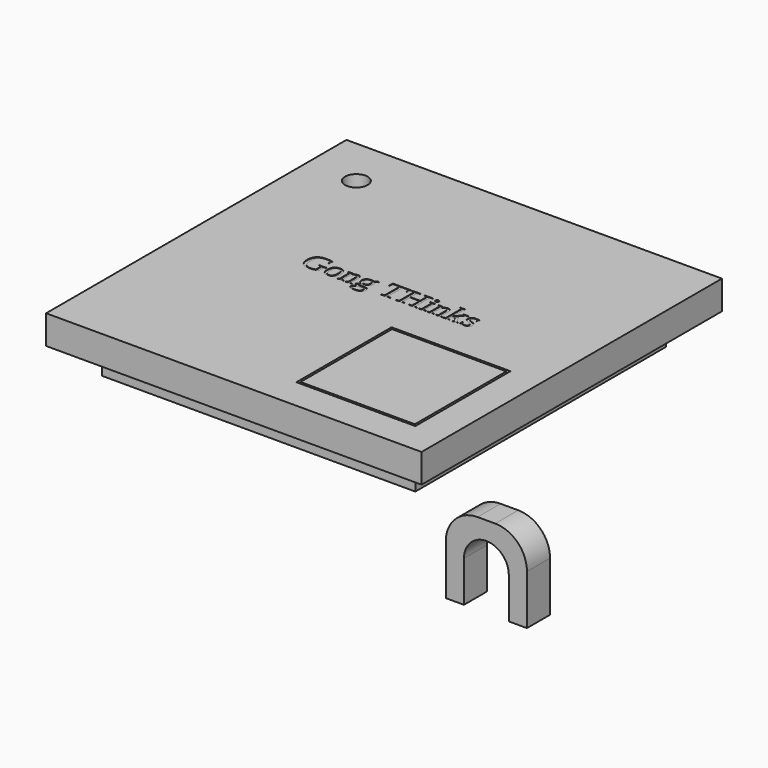
from build123d import *

# Parameters (mm, degrees)
F1_W        = 69
F1_H        = 69
F1_W_2      = 20.186291501
F1_H_2      = 20.186291501
F1_R        = 2.5
F2_DEPTH    = 6.35
F3_DEPTH    = 6.25
F4_W        = 9.8855943071
F4_H        = 4
F5_DEPTH    = 6.35
F6_R        = 7
F7_R        = 7
F8_R        = 5
F9_T1_DEPTH = 6.35
F0_W        = 82.7
F0_H        = 82.7
F0_W_2      = 26.19
F0_H_2      = 26.19
F10_DEPTH   = 6.35
F11_DEPTH   = 6.35
F0_W_3      = 25.19
F0_H_3      = 25.19
F12_DEPTH   = 6.35


# Not quite as in the source:
# - a fillet or chamfer that OpenCascade refuses, or shapes differently, is made with other operations: its cross-section is extruded or revolved along the edge and cut away or added


with BuildPart() as f2:
    # F1 (on Top) → F2 (new body)
    with BuildSketch(Plane.XY):
        Rectangle(F1_W, F1_H)
        with Locations((21.4068542495, -21.4068542495)):
            Rectangle(F1_W_2, F1_H_2, mode=Mode.SUBTRACT)
        with Locations((-30.5, 30.5)):
            Circle(F1_R, mode=Mode.SUBTRACT)
    extrude(amount=-F2_DEPTH)

    # F0 (on Top) → F3 (join)
    with BuildSketch(Plane.XY):
        with BuildLine():
            add(Edge.make_bspline(
                [(18.7366319096, 0.8951822917), (18.7366319096, 0.4210069444), (18.4366102082, 0.1763237847)],
                knots=[0, 0, 0, 1, 1, 1], degree=2))
            add(Edge.make_bspline(
                [(18.6774956249, 1.2548828125), (18.7366319096, 1.1089409722), (18.7366319096, 0.8951822917)],
                knots=[0, 0, 0, 1, 1, 1], degree=2))
            add(Edge.make_bspline(
                [(18.5114799999, 1.5142144097), (18.6183593401, 1.4008246528), (18.6774956249, 1.2548828125)],
                knots=[0, 0, 0, 1, 1, 1], degree=2))
            add(Edge.make_bspline(
                [(18.2521484026, 1.7057291667), (18.4046006596, 1.6276041667), (18.5114799999, 1.5142144097)],
                knots=[0, 0, 0, 1, 1, 1], degree=2))
            add(Edge.make_bspline(
                [(17.6016492707, 1.953125), (18.0996961457, 1.7838541667), (18.2521484026, 1.7057291667)],
                knots=[0, 0, 0, 1, 1, 1], degree=2))
            add(Edge.make_bspline(
                [(17.2061414582, 2.1733940972), (17.3368923263, 2.041015625), (17.6016492707, 1.953125)],
                knots=[0, 0, 0, 1, 1, 1], degree=2))
            add(Edge.make_bspline(
                [(17.0753905901, 2.4989149306), (17.0753905901, 2.3057725694), (17.2061414582, 2.1733940972)],
                knots=[0, 0, 0, 1, 1, 1], degree=2))
            add(Edge.make_bspline(
                [(17.2197048263, 2.8656684028), (17.0753905901, 2.7300347222), (17.0753905901, 2.4989149306)],
                knots=[0, 0, 0, 1, 1, 1], degree=2))
            add(Edge.make_bspline(
                [(17.6385416318, 3.0013020833), (17.3640190624, 3.0013020833), (17.2197048263, 2.8656684028)],
                knots=[0, 0, 0, 1, 1, 1], degree=2))
            add(Edge.make_bspline(
                [(18.2049478818, 2.841796875), (18.024826354, 3.0013020833), (17.6385416318, 3.0013020833)],
                knots=[0, 0, 0, 1, 1, 1], degree=2))
            Line((18.2049478818, 2.841796875), (18.347091979, 2.4717881944))
            Line((18.347091979, 2.4717881944), (18.5065971874, 2.4717881944))
            Line((18.5065971874, 2.4717881944), (18.5065971874, 3.1673177083))
            add(Edge.make_bspline(
                [(17.6320312151, 3.2725694444), (17.9814235763, 3.2725694444), (18.5065971874, 3.1673177083)],
                knots=[0, 0, 0, 1, 1, 1], degree=2))
            add(Edge.make_bspline(
                [(16.8572916318, 3.0300564236), (17.1437499651, 3.2725694444), (17.6320312151, 3.2725694444)],
                knots=[0, 0, 0, 1, 1, 1], degree=2))
            add(Edge.make_bspline(
                [(16.5708332985, 2.3665364583), (16.5708332985, 2.7875434028), (16.8572916318, 3.0300564236)],
                knots=[0, 0, 0, 1, 1, 1], degree=2))
            add(Edge.make_bspline(
                [(16.6554687151, 1.9618055556), (16.5708332985, 2.1299913194), (16.5708332985, 2.3665364583)],
                knots=[0, 0, 0, 1, 1, 1], degree=2))
            add(Edge.make_bspline(
                [(16.8958115971, 1.6786024306), (16.7401041318, 1.7936197917), (16.6554687151, 1.9618055556)],
                knots=[0, 0, 0, 1, 1, 1], degree=2))
            add(Edge.make_bspline(
                [(17.3944010068, 1.4518229167), (17.0515190624, 1.5635850694), (16.8958115971, 1.6786024306)],
                knots=[0, 0, 0, 1, 1, 1], degree=2))
            Line((17.3944010068, 1.4518229167), (17.6960503124, 1.3530815972))
            add(Edge.make_bspline(
                [(18.2147135068, 0.7628038194), (18.2147135068, 1.1762152778), (17.6960503124, 1.3530815972)],
                knots=[0, 0, 0, 1, 1, 1], degree=2))
            add(Edge.make_bspline(
                [(17.5571614235, 0.1996527778), (18.2147135068, 0.1996527778), (18.2147135068, 0.7628038194)],
                knots=[0, 0, 0, 1, 1, 1], degree=2))
            add(Edge.make_bspline(
                [(16.8963541318, 0.4307725694), (17.1502603818, 0.1996527778), (17.5571614235, 0.1996527778)],
                knots=[0, 0, 0, 1, 1, 1], degree=2))
            Line((16.8963541318, 0.4307725694), (16.7292534374, 0.8745659722))
            Line((16.7292534374, 0.8745659722), (16.5773437151, 0.8745659722))
            Line((16.5773437151, 0.8745659722), (16.5773437151, 0.0911458333))
            add(Edge.make_bspline(
                [(17.0265624651, -0.0189887153), (16.7401041318, 0.0303819444), (16.5773437151, 0.0911458333)],
                knots=[0, 0, 0, 1, 1, 1], degree=2))
            add(Edge.make_bspline(
                [(17.5506510068, -0.068359375), (17.3130207985, -0.068359375), (17.0265624651, -0.0189887153)],
                knots=[0, 0, 0, 1, 1, 1], degree=2))
            add(Edge.make_bspline(
                [(18.4366102082, 0.1763237847), (18.1365885068, -0.068359375), (17.5506510068, -0.068359375)],
                knots=[0, 0, 0, 1, 1, 1], degree=2))
        make_face()
        Polygon((15.2850260068, 2.9437934028), (13.9796874651, 1.5364583333), (13.9796874651, 4.8187934028), (12.9456162846, 4.8187934028), (12.9456162846, 4.6657986111), (13.4165364235, 4.5844184028), (13.4165364235, 0.2376302083), (13.0128905901, 0.1529947917), (13.0128905901, 0), (14.3193142013, 0), (14.3193142013, 0.1529947917), (13.9796874651, 0.2376302083), (13.9796874651, 1.1534288194), (14.3963541318, 1.6102430556), (15.2720051735, 0.2376302083), (14.9801214929, 0.1529947917), (14.9801214929, 0), (16.2854600346, 0), (16.2854600346, 0.1529947917), (15.9393228818, 0.2311197917), (14.772873229, 2.0279947917), (15.6821614235, 2.9568142361), (16.0782117707, 3.0349392361), (16.0782117707, 3.1879340278), (14.9529947568, 3.1879340278), (14.9529947568, 3.0349392361), align=None)
        with BuildLine():
            add(Edge.make_bspline(
                [(10.4401909374, 2.9296875), (10.700607604, 3.0794270833), (10.9957464929, 3.1759982639)],
                knots=[0, 0, 0, 1, 1, 1], degree=2))
            Line((10.4401909374, 2.9296875), (10.4087239235, 3.1879340278))
            Line((10.4087239235, 3.1879340278), (9.5005207985, 3.1879340278))
            Line((9.5005207985, 3.1879340278), (9.5005207985, 3.0349392361))
            Line((9.5005207985, 3.0349392361), (9.8835503124, 2.9503038194))
            Line((9.8835503124, 2.9503038194), (9.8835503124, 0.2376302083))
            Line((9.8835503124, 0.2376302083), (9.5005207985, 0.1529947917))
            Line((9.5005207985, 0.1529947917), (9.5005207985, 0))
            Line((9.5005207985, 0), (10.8774739235, 0))
            Line((10.8774739235, 0), (10.8774739235, 0.1529947917))
            Line((10.8774739235, 0.1529947917), (10.446701354, 0.2376302083))
            Line((10.446701354, 0.2376302083), (10.446701354, 2.7766927083))
            add(Edge.make_bspline(
                [(11.1953992707, 2.8754340278), (10.8904947568, 2.8754340278), (10.446701354, 2.7766927083)],
                knots=[0, 0, 0, 1, 1, 1], degree=2))
            add(Edge.make_bspline(
                [(11.6212890276, 2.7143012153), (11.4840277429, 2.8754340278), (11.1953992707, 2.8754340278)],
                knots=[0, 0, 0, 1, 1, 1], degree=2))
            add(Edge.make_bspline(
                [(11.7585503124, 2.2721354167), (11.7585503124, 2.5531684028), (11.6212890276, 2.7143012153)],
                knots=[0, 0, 0, 1, 1, 1], degree=2))
            Line((11.7585503124, 2.2721354167), (11.7585503124, 0.2376302083))
            Line((11.7585503124, 0.2376302083), (11.335373229, 0.1529947917))
            Line((11.335373229, 0.1529947917), (11.335373229, 0))
            Line((11.335373229, 0), (12.7079860763, 0))
            Line((12.7079860763, 0), (12.7079860763, 0.1529947917))
            Line((12.7079860763, 0.1529947917), (12.321701354, 0.2376302083))
            Line((12.321701354, 0.2376302083), (12.321701354, 2.3328993056))
            add(Edge.make_bspline(
                [(12.1111978818, 3.0316840278), (12.321701354, 2.7907986111), (12.321701354, 2.3328993056)],
                knots=[0, 0, 0, 1, 1, 1], degree=2))
            add(Edge.make_bspline(
                [(11.4872829513, 3.2725694444), (11.9006944096, 3.2725694444), (12.1111978818, 3.0316840278)],
                knots=[0, 0, 0, 1, 1, 1], degree=2))
            add(Edge.make_bspline(
                [(10.9957464929, 3.1759982639), (11.2908853818, 3.2725694444), (11.4872829513, 3.2725694444)],
                knots=[0, 0, 0, 1, 1, 1], degree=2))
        make_face()
        Polygon((9.2086371179, 0.1529947917), (8.6628471874, 0.2376302083), (8.6628471874, 3.1879340278), (7.6493923263, 3.1879340278), (7.6493923263, 3.0349392361), (8.0996961457, 2.9503038194), (8.0996961457, 0.2376302083), (7.5571614235, 0.1529947917), (7.5571614235, 0), (9.2086371179, 0), align=None)
        Polygon((2.5962239235, 0.1801215278), (2.5962239235, 0), (4.4180555207, 0), (4.4180555207, 0.1801215278), (3.8342881596, 0.2712673611), (3.8342881596, 2.1875), (5.974045104, 2.1875), (5.974045104, 0.2712673611), (5.3902777429, 0.1801215278), (5.3902777429, 0), (7.2077690624, 0), (7.2077690624, 0.1801215278), (6.6250867707, 0.2712673611), (6.6250867707, 4.2795138889), (7.2077690624, 4.3674045139), (7.2077690624, 4.5475260417), (5.3902777429, 4.5475260417), (5.3902777429, 4.3674045139), (5.974045104, 4.2795138889), (5.974045104, 2.4924045139), (3.8342881596, 2.4924045139), (3.8342881596, 4.2795138889), (4.4180555207, 4.3674045139), (4.4180555207, 4.5475260417), (2.5962239235, 4.5475260417), (2.5962239235, 4.3674045139), (3.1799912846, 4.2795138889), (3.1799912846, 0.2712673611), align=None)
        with BuildLine():
            Line((-0.7772569793, 0.1801215278), (-0.7772569793, 0))
            Line((-0.7772569793, 0), (1.3223523957, 0))
            Line((1.3223523957, 0), (1.3223523957, 0.1801215278))
            Line((1.3223523957, 0.1801215278), (0.5996961457, 0.2712673611))
            Line((0.5996961457, 0.2712673611), (0.5996961457, 4.2491319444))
            Line((0.5996961457, 4.2491319444), (0.7657117707, 4.2491319444))
            add(Edge.make_bspline(
                [(1.5154947568, 4.2301432292), (1.1726128124, 4.2491319444), (0.7657117707, 4.2491319444)],
                knots=[0, 0, 0, 1, 1, 1], degree=2))
            add(Edge.make_bspline(
                [(1.9592881596, 4.1872829861), (1.8583767013, 4.2111545139), (1.5154947568, 4.2301432292)],
                knots=[0, 0, 0, 1, 1, 1], degree=2))
            Line((1.9592881596, 4.1872829861), (2.0515190624, 3.4787326389))
            Line((2.0515190624, 3.4787326389), (2.2815537846, 3.4787326389))
            Line((2.2815537846, 3.4787326389), (2.2815537846, 4.5475260417))
            Line((2.2815537846, 4.5475260417), (-1.7190972571, 4.5475260417))
            Line((-1.7190972571, 4.5475260417), (-1.7190972571, 3.4787326389))
            Line((-1.7190972571, 3.4787326389), (-1.4923177432, 3.4787326389))
            Line((-1.4923177432, 3.4787326389), (-1.4011719099, 4.1872829861))
            add(Edge.make_bspline(
                [(-0.227126771, 4.2556423611), (-1.0854167015, 4.2556423611), (-1.4011719099, 4.1872829861)],
                knots=[0, 0, 0, 1, 1, 1], degree=2))
            Line((-0.227126771, 4.2556423611), (-0.0546007293, 4.2556423611))
            Line((-0.0546007293, 4.2556423611), (-0.0546007293, 0.2712673611))
            Line((-0.0546007293, 0.2712673611), (-0.7772569793, 0.1801215278))
        make_face()
        with BuildLine():
            add(Edge.make_bspline(
                [(-4.1029948265, 2.1799045139), (-4.1029948265, 1.630859375), (-4.4317708682, 1.3492838542)],
                knots=[0, 0, 0, 1, 1, 1], degree=2))
            add(Edge.make_bspline(
                [(-4.3308594099, 2.9296875), (-4.1029948265, 2.67578125), (-4.1029948265, 2.1799045139)],
                knots=[0, 0, 0, 1, 1, 1], degree=2))
            Line((-4.3308594099, 2.9296875), (-3.8588542015, 3.41796875))
            Line((-3.8588542015, 3.41796875), (-3.9782118404, 3.5633680556))
            Line((-3.9782118404, 3.5633680556), (-4.7269097571, 3.1879340278))
            add(Edge.make_bspline(
                [(-5.0291015974, 3.2470703125), (-4.8321614932, 3.2215711806), (-4.7269097571, 3.1879340278)],
                knots=[0, 0, 0, 1, 1, 1], degree=2))
            add(Edge.make_bspline(
                [(-5.3508246876, 3.2725694444), (-5.2260417015, 3.2725694444), (-5.0291015974, 3.2470703125)],
                knots=[0, 0, 0, 1, 1, 1], degree=2))
            add(Edge.make_bspline(
                [(-6.3121962154, 2.9877387153), (-5.9812500349, 3.2725694444), (-5.3508246876, 3.2725694444)],
                knots=[0, 0, 0, 1, 1, 1], degree=2))
            add(Edge.make_bspline(
                [(-6.643142396, 2.1799045139), (-6.643142396, 2.7029079861), (-6.3121962154, 2.9877387153)],
                knots=[0, 0, 0, 1, 1, 1], degree=2))
            add(Edge.make_bspline(
                [(-6.1071180904, 1.1935763889), (-6.643142396, 1.4442274306), (-6.643142396, 2.1799045139)],
                knots=[0, 0, 0, 1, 1, 1], degree=2))
            Line((-6.1071180904, 1.1935763889), (-6.643142396, 0.5902777778))
            add(Edge.make_bspline(
                [(-6.5107639237, 0.2544487847), (-6.643142396, 0.41015625), (-6.643142396, 0.5902777778)],
                knots=[0, 0, 0, 1, 1, 1], degree=2))
            add(Edge.make_bspline(
                [(-6.1852430904, 0.0336371528), (-6.3783854515, 0.0987413194), (-6.5107639237, 0.2544487847)],
                knots=[0, 0, 0, 1, 1, 1], degree=2))
            add(Edge.make_bspline(
                [(-6.6328342362, -0.3743489583), (-6.5107639237, -0.1996527778), (-6.1852430904, 0.0336371528)],
                knots=[0, 0, 0, 1, 1, 1], degree=2))
            add(Edge.make_bspline(
                [(-6.7549045487, -0.7291666667), (-6.7549045487, -0.5490451389), (-6.6328342362, -0.3743489583)],
                knots=[0, 0, 0, 1, 1, 1], degree=2))
            add(Edge.make_bspline(
                [(-6.4141927432, -1.298828125), (-6.7549045487, -1.0991753472), (-6.7549045487, -0.7291666667)],
                knots=[0, 0, 0, 1, 1, 1], degree=2))
            add(Edge.make_bspline(
                [(-5.422439271, -1.4984809028), (-6.0734809376, -1.4984809028), (-6.4141927432, -1.298828125)],
                knots=[0, 0, 0, 1, 1, 1], degree=2))
            add(Edge.make_bspline(
                [(-4.4930772918, -1.3547092014), (-4.8766493404, -1.4984809028), (-5.422439271, -1.4984809028)],
                knots=[0, 0, 0, 1, 1, 1], degree=2))
            add(Edge.make_bspline(
                [(-3.9114800696, -0.9461805556), (-4.1095052432, -1.2109375), (-4.4930772918, -1.3547092014)],
                knots=[0, 0, 0, 1, 1, 1], degree=2))
            add(Edge.make_bspline(
                [(-3.713454896, -0.3255208333), (-3.713454896, -0.6814236111), (-3.9114800696, -0.9461805556)],
                knots=[0, 0, 0, 1, 1, 1], degree=2))
            add(Edge.make_bspline(
                [(-3.9624783335, 0.2918836806), (-3.713454896, 0.068359375), (-3.713454896, -0.3255208333)],
                knots=[0, 0, 0, 1, 1, 1], degree=2))
            add(Edge.make_bspline(
                [(-4.7269097571, 0.5154079861), (-4.211501771, 0.5154079861), (-3.9624783335, 0.2918836806)],
                knots=[0, 0, 0, 1, 1, 1], degree=2))
            Line((-4.7269097571, 0.5154079861), (-5.6698351043, 0.5154079861))
            add(Edge.make_bspline(
                [(-5.9752821529, 0.56640625), (-5.8532118404, 0.5154079861), (-5.6698351043, 0.5154079861)],
                knots=[0, 0, 0, 1, 1, 1], degree=2))
            add(Edge.make_bspline(
                [(-6.1071180904, 0.6749131944), (-6.0973524654, 0.6174045139), (-5.9752821529, 0.56640625)],
                knots=[0, 0, 0, 1, 1, 1], degree=2))
            Line((-6.1071180904, 0.6749131944), (-5.8933594099, 1.1187065972))
            add(Edge.make_bspline(
                [(-5.3779514237, 1.0677083333), (-5.6557292015, 1.0677083333), (-5.8933594099, 1.1187065972)],
                knots=[0, 0, 0, 1, 1, 1], degree=2))
            add(Edge.make_bspline(
                [(-4.4317708682, 1.3492838542), (-4.7605469099, 1.0677083333), (-5.3779514237, 1.0677083333)],
                knots=[0, 0, 0, 1, 1, 1], degree=2))
        make_face()
        with BuildLine():
            add(Edge.make_bspline(
                [(-4.2418837154, -0.4307725694), (-4.2418837154, -0.2376302083), (-4.3606988196, -0.1291232639)],
                knots=[0, 0, 0, 1, 1, 1], degree=2))
            add(Edge.make_bspline(
                [(-4.5489583682, -1.0172526042), (-4.2418837154, -0.8072916667), (-4.2418837154, -0.4307725694)],
                knots=[0, 0, 0, 1, 1, 1], degree=2))
            add(Edge.make_bspline(
                [(-5.422439271, -1.2272135417), (-4.856033021, -1.2272135417), (-4.5489583682, -1.0172526042)],
                knots=[0, 0, 0, 1, 1, 1], degree=2))
            add(Edge.make_bspline(
                [(-6.0664279862, -1.1002604167), (-5.8564670487, -1.2272135417), (-5.422439271, -1.2272135417)],
                knots=[0, 0, 0, 1, 1, 1], degree=2))
            add(Edge.make_bspline(
                [(-6.2763889237, -0.6814236111), (-6.2763889237, -0.9733072917), (-6.0664279862, -1.1002604167)],
                knots=[0, 0, 0, 1, 1, 1], degree=2))
            add(Edge.make_bspline(
                [(-6.1868706946, -0.3304036458), (-6.2763889237, -0.5186631944), (-6.2763889237, -0.6814236111)],
                knots=[0, 0, 0, 1, 1, 1], degree=2))
            add(Edge.make_bspline(
                [(-5.9541232987, -0.0206163194), (-6.0973524654, -0.1421440972), (-6.1868706946, -0.3304036458)],
                knots=[0, 0, 0, 1, 1, 1], degree=2))
            Line((-5.9541232987, -0.0206163194), (-4.7203993404, -0.0206163194))
            add(Edge.make_bspline(
                [(-4.3606988196, -0.1291232639), (-4.4795139237, -0.0206163194), (-4.7203993404, -0.0206163194)],
                knots=[0, 0, 0, 1, 1, 1], degree=2))
        make_face(mode=Mode.SUBTRACT)
        with BuildLine():
            add(Edge.make_bspline(
                [(-5.3714410071, 1.3259548611), (-5.0014323265, 1.3259548611), (-4.8473524654, 1.5380859375)],
                knots=[0, 0, 0, 1, 1, 1], degree=2))
            add(Edge.make_bspline(
                [(-5.8901042015, 1.5294053819), (-5.7273437849, 1.3259548611), (-5.3714410071, 1.3259548611)],
                knots=[0, 0, 0, 1, 1, 1], degree=2))
            add(Edge.make_bspline(
                [(-6.0528646182, 2.1804470486), (-6.0528646182, 1.7328559028), (-5.8901042015, 1.5294053819)],
                knots=[0, 0, 0, 1, 1, 1], degree=2))
            add(Edge.make_bspline(
                [(-5.8868489932, 2.8211805556), (-6.0528646182, 2.6280381944), (-6.0528646182, 2.1804470486)],
                knots=[0, 0, 0, 1, 1, 1], degree=2))
            add(Edge.make_bspline(
                [(-5.3649305904, 3.0143229167), (-5.7208333682, 3.0143229167), (-5.8868489932, 2.8211805556)],
                knots=[0, 0, 0, 1, 1, 1], degree=2))
            add(Edge.make_bspline(
                [(-4.8527778126, 2.8228081597), (-5.012283021, 3.0143229167), (-5.3649305904, 3.0143229167)],
                knots=[0, 0, 0, 1, 1, 1], degree=2))
            add(Edge.make_bspline(
                [(-4.6932726043, 2.1799045139), (-4.6932726043, 2.6312934028), (-4.8527778126, 2.8228081597)],
                knots=[0, 0, 0, 1, 1, 1], degree=2))
            add(Edge.make_bspline(
                [(-4.8473524654, 1.5380859375), (-4.6932726043, 1.7502170139), (-4.6932726043, 2.1799045139)],
                knots=[0, 0, 0, 1, 1, 1], degree=2))
        make_face(mode=Mode.SUBTRACT)
        with BuildLine():
            add(Edge.make_bspline(
                [(-9.426345521, 2.9296875), (-9.1659288543, 3.0794270833), (-8.8707899654, 3.1759982639)],
                knots=[0, 0, 0, 1, 1, 1], degree=2))
            Line((-9.426345521, 2.9296875), (-9.4578125349, 3.1879340278))
            Line((-9.4578125349, 3.1879340278), (-10.3660156599, 3.1879340278))
            Line((-10.3660156599, 3.1879340278), (-10.3660156599, 3.0349392361))
            Line((-10.3660156599, 3.0349392361), (-9.982986146, 2.9503038194))
            Line((-9.982986146, 2.9503038194), (-9.982986146, 0.2376302083))
            Line((-9.982986146, 0.2376302083), (-10.3660156599, 0.1529947917))
            Line((-10.3660156599, 0.1529947917), (-10.3660156599, 0))
            Line((-10.3660156599, 0), (-8.9890625349, 0))
            Line((-8.9890625349, 0), (-8.9890625349, 0.1529947917))
            Line((-8.9890625349, 0.1529947917), (-9.4198351043, 0.2376302083))
            Line((-9.4198351043, 0.2376302083), (-9.4198351043, 2.7766927083))
            add(Edge.make_bspline(
                [(-8.6711371876, 2.8754340278), (-8.9760417015, 2.8754340278), (-9.4198351043, 2.7766927083)],
                knots=[0, 0, 0, 1, 1, 1], degree=2))
            add(Edge.make_bspline(
                [(-8.2452474307, 2.7143012153), (-8.3825087154, 2.8754340278), (-8.6711371876, 2.8754340278)],
                knots=[0, 0, 0, 1, 1, 1], degree=2))
            add(Edge.make_bspline(
                [(-8.107986146, 2.2721354167), (-8.107986146, 2.5531684028), (-8.2452474307, 2.7143012153)],
                knots=[0, 0, 0, 1, 1, 1], degree=2))
            Line((-8.107986146, 2.2721354167), (-8.107986146, 0.2376302083))
            Line((-8.107986146, 0.2376302083), (-8.5311632293, 0.1529947917))
            Line((-8.5311632293, 0.1529947917), (-8.5311632293, 0))
            Line((-8.5311632293, 0), (-7.1585503821, 0))
            Line((-7.1585503821, 0), (-7.1585503821, 0.1529947917))
            Line((-7.1585503821, 0.1529947917), (-7.5448351043, 0.2376302083))
            Line((-7.5448351043, 0.2376302083), (-7.5448351043, 2.3328993056))
            add(Edge.make_bspline(
                [(-7.7553385765, 3.0316840278), (-7.5448351043, 2.7907986111), (-7.5448351043, 2.3328993056)],
                knots=[0, 0, 0, 1, 1, 1], degree=2))
            add(Edge.make_bspline(
                [(-8.3792535071, 3.2725694444), (-7.9658420487, 3.2725694444), (-7.7553385765, 3.0316840278)],
                knots=[0, 0, 0, 1, 1, 1], degree=2))
            add(Edge.make_bspline(
                [(-8.8707899654, 3.1759982639), (-8.5756510765, 3.2725694444), (-8.3792535071, 3.2725694444)],
                knots=[0, 0, 0, 1, 1, 1], degree=2))
        make_face()
        with BuildLine():
            add(Edge.make_bspline(
                [(-10.7902778126, 1.6102430556), (-10.7902778126, -0.068359375), (-12.2822482987, -0.068359375)],
                knots=[0, 0, 0, 1, 1, 1], degree=2))
            add(Edge.make_bspline(
                [(-11.1597439585, 2.8537326389), (-10.7902778126, 2.4348958333), (-10.7902778126, 1.6102430556)],
                knots=[0, 0, 0, 1, 1, 1], degree=2))
            add(Edge.make_bspline(
                [(-12.2551215626, 3.2725694444), (-11.5292101043, 3.2725694444), (-11.1597439585, 2.8537326389)],
                knots=[0, 0, 0, 1, 1, 1], degree=2))
            add(Edge.make_bspline(
                [(-13.3667752085, 2.8450520833), (-13.000564271, 3.2725694444), (-12.2551215626, 3.2725694444)],
                knots=[0, 0, 0, 1, 1, 1], degree=2))
            add(Edge.make_bspline(
                [(-13.732986146, 1.6102430556), (-13.732986146, 2.4175347222), (-13.3667752085, 2.8450520833)],
                knots=[0, 0, 0, 1, 1, 1], degree=2))
            add(Edge.make_bspline(
                [(-13.3667752085, 0.3624131944), (-13.732986146, 0.7931857639), (-13.732986146, 1.6102430556)],
                knots=[0, 0, 0, 1, 1, 1], degree=2))
            add(Edge.make_bspline(
                [(-12.2822482987, -0.068359375), (-13.000564271, -0.068359375), (-13.3667752085, 0.3624131944)],
                knots=[0, 0, 0, 1, 1, 1], degree=2))
        make_face()
        with BuildLine():
            add(Edge.make_bspline(
                [(-11.4000868404, 1.6102430556), (-11.4000868404, 2.3426649306), (-11.613845521, 2.6719835069)],
                knots=[0, 0, 0, 1, 1, 1], degree=2))
            add(Edge.make_bspline(
                [(-11.6171007293, 0.5322265625), (-11.4000868404, 0.8648003472), (-11.4000868404, 1.6102430556)],
                knots=[0, 0, 0, 1, 1, 1], degree=2))
            add(Edge.make_bspline(
                [(-12.2822482987, 0.1996527778), (-11.8341146182, 0.1996527778), (-11.6171007293, 0.5322265625)],
                knots=[0, 0, 0, 1, 1, 1], degree=2))
            add(Edge.make_bspline(
                [(-12.9213542015, 0.5202907986), (-12.7195312849, 0.1996527778), (-12.2822482987, 0.1996527778)],
                knots=[0, 0, 0, 1, 1, 1], degree=2))
            add(Edge.make_bspline(
                [(-13.1231771182, 1.6102430556), (-13.1231771182, 0.8409288194), (-12.9213542015, 0.5202907986)],
                knots=[0, 0, 0, 1, 1, 1], degree=2))
            add(Edge.make_bspline(
                [(-12.9246094099, 2.685546875), (-13.1231771182, 2.3697916667), (-13.1231771182, 1.6102430556)],
                knots=[0, 0, 0, 1, 1, 1], degree=2))
            add(Edge.make_bspline(
                [(-12.2822482987, 3.0013020833), (-12.7260417015, 3.0013020833), (-12.9246094099, 2.685546875)],
                knots=[0, 0, 0, 1, 1, 1], degree=2))
            add(Edge.make_bspline(
                [(-11.613845521, 2.6719835069), (-11.8276042015, 3.0013020833), (-12.2822482987, 3.0013020833)],
                knots=[0, 0, 0, 1, 1, 1], degree=2))
        make_face(mode=Mode.SUBTRACT)
        with BuildLine():
            add(Edge.make_bspline(
                [(-14.6585503821, 0.2376302083), (-15.0524305904, 0.1085069444), (-15.4761502085, 0.0200737847)],
                knots=[0, 0, 0, 1, 1, 1], degree=2))
            Line((-14.6585503821, 0.2376302083), (-14.6585503821, 1.7154947917))
            Line((-14.6585503821, 1.7154947917), (-14.2147569793, 1.8044704861))
            Line((-14.2147569793, 1.8044704861), (-14.2147569793, 1.9867621528))
            Line((-14.2147569793, 1.9867621528), (-15.8933594099, 1.9867621528))
            Line((-15.8933594099, 1.9867621528), (-15.8933594099, 1.8044704861))
            Line((-15.8933594099, 1.8044704861), (-15.3095920487, 1.7154947917))
            Line((-15.3095920487, 1.7154947917), (-15.3095920487, 0.4242621528))
            add(Edge.make_bspline(
                [(-15.7843099307, 0.2609592014), (-15.4723524654, 0.3287760417), (-15.3095920487, 0.4242621528)],
                knots=[0, 0, 0, 1, 1, 1], degree=2))
            add(Edge.make_bspline(
                [(-16.3816406599, 0.1931423611), (-16.096267396, 0.1931423611), (-15.7843099307, 0.2609592014)],
                knots=[0, 0, 0, 1, 1, 1], degree=2))
            add(Edge.make_bspline(
                [(-17.6055989932, 0.7101779514), (-17.1921875349, 0.1931423611), (-16.3816406599, 0.1931423611)],
                knots=[0, 0, 0, 1, 1, 1], degree=2))
            add(Edge.make_bspline(
                [(-18.0190104515, 2.2276475694), (-18.0190104515, 1.2272135417), (-17.6055989932, 0.7101779514)],
                knots=[0, 0, 0, 1, 1, 1], degree=2))
            add(Edge.make_bspline(
                [(-17.6175347571, 3.8096788194), (-18.0190104515, 3.2921006944), (-18.0190104515, 2.2276475694)],
                knots=[0, 0, 0, 1, 1, 1], degree=2))
            add(Edge.make_bspline(
                [(-16.3480035071, 4.3272569444), (-17.2160590626, 4.3272569444), (-17.6175347571, 3.8096788194)],
                knots=[0, 0, 0, 1, 1, 1], degree=2))
            add(Edge.make_bspline(
                [(-15.6573568057, 4.2371961806), (-15.9845052432, 4.3272569444), (-16.3480035071, 4.3272569444)],
                knots=[0, 0, 0, 1, 1, 1], degree=2))
            add(Edge.make_bspline(
                [(-15.0969184376, 3.9811197917), (-15.3302083682, 4.1471354167), (-15.6573568057, 4.2371961806)],
                knots=[0, 0, 0, 1, 1, 1], degree=2))
            Line((-15.0969184376, 3.9811197917), (-15.0046875349, 3.41796875))
            Line((-15.0046875349, 3.41796875), (-14.777908021, 3.41796875))
            Line((-14.777908021, 3.41796875), (-14.777908021, 4.39453125))
            add(Edge.make_bspline(
                [(-16.3751302432, 4.5985243056), (-15.5472222571, 4.5985243056), (-14.777908021, 4.39453125)],
                knots=[0, 0, 0, 1, 1, 1], degree=2))
            add(Edge.make_bspline(
                [(-18.1291450001, 4.0066189236), (-17.5307292015, 4.5985243056), (-16.3751302432, 4.5985243056)],
                knots=[0, 0, 0, 1, 1, 1], degree=2))
            add(Edge.make_bspline(
                [(-18.7275607987, 2.2211371528), (-18.7275607987, 3.4147135417), (-18.1291450001, 4.0066189236)],
                knots=[0, 0, 0, 1, 1, 1], degree=2))
            add(Edge.make_bspline(
                [(-18.1106988196, 0.5289713542), (-18.7275607987, 1.1263020833), (-18.7275607987, 2.2211371528)],
                knots=[0, 0, 0, 1, 1, 1], degree=2))
            add(Edge.make_bspline(
                [(-16.3881510765, -0.068359375), (-17.4938368404, -0.068359375), (-18.1106988196, 0.5289713542)],
                knots=[0, 0, 0, 1, 1, 1], degree=2))
            add(Edge.make_bspline(
                [(-15.4761502085, 0.0200737847), (-15.8998698265, -0.068359375), (-16.3881510765, -0.068359375)],
                knots=[0, 0, 0, 1, 1, 1], degree=2))
        make_face()
    extrude(amount=F3_DEPTH)


with BuildPart() as f5:
    # F4 (on Front) → F5 (new body)
    with BuildSketch(Plane.XZ):
        with Locations((27.6252044371, -27.5937509686)):
            Rectangle(F4_W, F4_H)
        Polygon((36.5680015907, -25.5937509686), (32.5680015907, -25.5937509686), (32.5680015907, -29.5937509686), (32.5680015907, -43.5937509686), (36.5680015907, -43.5937509686), align=None)
        Polygon((22.6824072836, -25.5937509686), (18.6824072836, -25.5937509686), (18.6824072836, -43.5937509686), (22.6824072836, -43.5937509686), (22.6824072836, -29.5937509686), align=None)
    extrude(amount=F5_DEPTH)

    # F6
    f6_edges = [f5.edges().sort_by_distance(p)[0] for p in [
        (36.568002, -3.175, -25.593751),
    ]]
    fillet(f6_edges, radius=F6_R)

    # F7
    f7_edges = [f5.edges().sort_by_distance(p)[0] for p in [
        (18.682407, -3.175, -25.593751),
    ]]
    fillet(f7_edges, radius=F7_R)

    # F8
    f8_edges = [f5.edges().sort_by_distance(p)[0] for p in [
        (32.568002, -3.175, -29.593751),
    ]]
    fillet(f8_edges, radius=F8_R)

    # F9: fillet of radius 5 on 1 edges, made by hand

    # F9_s2 → F9_t1 (join)
    with BuildSketch(Plane.XZ):
        with BuildLine():
            ThreePointArc((27.5680015907, -29.5937509686), (24.1066536243, -31.0975906083), (22.6824072836, -34.592441931))
            Line((22.6824072836, -34.592441931), (22.6824072836, -29.5937509686))
            Line((22.6824072836, -29.5937509686), (27.5680015907, -29.5937509686))
        make_face()
    extrude(amount=F9_T1_DEPTH)


with BuildPart() as f10:
    # F0 (on Top) → F10 (new body)
    with BuildSketch(Plane.XY):
        Rectangle(F0_W, F0_H)
        with Locations((21.405, -21.405)):
            Rectangle(F0_W_2, F0_H_2, mode=Mode.SUBTRACT)
        with BuildLine():
            Line((-14.6585503821, 1.7154947917), (-14.6585503821, 0.2376302083))
            add(Edge.make_bspline(
                [(-14.6585503821, 0.2376302083), (-15.0524305904, 0.1085069444), (-15.4761502085, 0.0200737847)],
                knots=[0, 0, 0, 1, 1, 1], degree=2))
            add(Edge.make_bspline(
                [(-15.4761502085, 0.0200737847), (-15.8998698265, -0.068359375), (-16.3881510765, -0.068359375)],
                knots=[0, 0, 0, 1, 1, 1], degree=2))
            add(Edge.make_bspline(
                [(-16.3881510765, -0.068359375), (-17.4938368404, -0.068359375), (-18.1106988196, 0.5289713542)],
                knots=[0, 0, 0, 1, 1, 1], degree=2))
            add(Edge.make_bspline(
                [(-18.1106988196, 0.5289713542), (-18.7275607987, 1.1263020833), (-18.7275607987, 2.2211371528)],
                knots=[0, 0, 0, 1, 1, 1], degree=2))
            add(Edge.make_bspline(
                [(-18.7275607987, 2.2211371528), (-18.7275607987, 3.4147135417), (-18.1291450001, 4.0066189236)],
                knots=[0, 0, 0, 1, 1, 1], degree=2))
            add(Edge.make_bspline(
                [(-18.1291450001, 4.0066189236), (-17.5307292015, 4.5985243056), (-16.3751302432, 4.5985243056)],
                knots=[0, 0, 0, 1, 1, 1], degree=2))
            add(Edge.make_bspline(
                [(-16.3751302432, 4.5985243056), (-15.5472222571, 4.5985243056), (-14.777908021, 4.39453125)],
                knots=[0, 0, 0, 1, 1, 1], degree=2))
            Line((-14.777908021, 4.39453125), (-14.777908021, 3.41796875))
            Line((-14.777908021, 3.41796875), (-15.0046875349, 3.41796875))
            Line((-15.0046875349, 3.41796875), (-15.0969184376, 3.9811197917))
            add(Edge.make_bspline(
                [(-15.0969184376, 3.9811197917), (-15.3302083682, 4.1471354167), (-15.6573568057, 4.2371961806)],
                knots=[0, 0, 0, 1, 1, 1], degree=2))
            add(Edge.make_bspline(
                [(-15.6573568057, 4.2371961806), (-15.9845052432, 4.3272569444), (-16.3480035071, 4.3272569444)],
                knots=[0, 0, 0, 1, 1, 1], degree=2))
            add(Edge.make_bspline(
                [(-16.3480035071, 4.3272569444), (-17.2160590626, 4.3272569444), (-17.6175347571, 3.8096788194)],
                knots=[0, 0, 0, 1, 1, 1], degree=2))
            add(Edge.make_bspline(
                [(-17.6175347571, 3.8096788194), (-18.0190104515, 3.2921006944), (-18.0190104515, 2.2276475694)],
                knots=[0, 0, 0, 1, 1, 1], degree=2))
            add(Edge.make_bspline(
                [(-18.0190104515, 2.2276475694), (-18.0190104515, 1.2272135417), (-17.6055989932, 0.7101779514)],
                knots=[0, 0, 0, 1, 1, 1], degree=2))
            add(Edge.make_bspline(
                [(-17.6055989932, 0.7101779514), (-17.1921875349, 0.1931423611), (-16.3816406599, 0.1931423611)],
                knots=[0, 0, 0, 1, 1, 1], degree=2))
            add(Edge.make_bspline(
                [(-16.3816406599, 0.1931423611), (-16.096267396, 0.1931423611), (-15.7843099307, 0.2609592014)],
                knots=[0, 0, 0, 1, 1, 1], degree=2))
            add(Edge.make_bspline(
                [(-15.7843099307, 0.2609592014), (-15.4723524654, 0.3287760417), (-15.3095920487, 0.4242621528)],
                knots=[0, 0, 0, 1, 1, 1], degree=2))
            Line((-15.3095920487, 0.4242621528), (-15.3095920487, 1.7154947917))
            Line((-15.3095920487, 1.7154947917), (-15.8933594099, 1.8044704861))
            Line((-15.8933594099, 1.8044704861), (-15.8933594099, 1.9867621528))
            Line((-15.8933594099, 1.9867621528), (-14.2147569793, 1.9867621528))
            Line((-14.2147569793, 1.9867621528), (-14.2147569793, 1.8044704861))
            Line((-14.2147569793, 1.8044704861), (-14.6585503821, 1.7154947917))
        make_face(mode=Mode.SUBTRACT)
        with BuildLine():
            add(Edge.make_bspline(
                [(-11.1597439585, 2.8537326389), (-10.7902778126, 2.4348958333), (-10.7902778126, 1.6102430556)],
                knots=[0, 0, 0, 1, 1, 1], degree=2))
            add(Edge.make_bspline(
                [(-10.7902778126, 1.6102430556), (-10.7902778126, -0.068359375), (-12.2822482987, -0.068359375)],
                knots=[0, 0, 0, 1, 1, 1], degree=2))
            add(Edge.make_bspline(
                [(-12.2822482987, -0.068359375), (-13.000564271, -0.068359375), (-13.3667752085, 0.3624131944)],
                knots=[0, 0, 0, 1, 1, 1], degree=2))
            add(Edge.make_bspline(
                [(-13.3667752085, 0.3624131944), (-13.732986146, 0.7931857639), (-13.732986146, 1.6102430556)],
                knots=[0, 0, 0, 1, 1, 1], degree=2))
            add(Edge.make_bspline(
                [(-13.732986146, 1.6102430556), (-13.732986146, 2.4175347222), (-13.3667752085, 2.8450520833)],
                knots=[0, 0, 0, 1, 1, 1], degree=2))
            add(Edge.make_bspline(
                [(-13.3667752085, 2.8450520833), (-13.000564271, 3.2725694444), (-12.2551215626, 3.2725694444)],
                knots=[0, 0, 0, 1, 1, 1], degree=2))
            add(Edge.make_bspline(
                [(-12.2551215626, 3.2725694444), (-11.5292101043, 3.2725694444), (-11.1597439585, 2.8537326389)],
                knots=[0, 0, 0, 1, 1, 1], degree=2))
        make_face(mode=Mode.SUBTRACT)
        with BuildLine():
            Line((-9.4578125349, 3.1879340278), (-9.426345521, 2.9296875))
            add(Edge.make_bspline(
                [(-9.426345521, 2.9296875), (-9.1659288543, 3.0794270833), (-8.8707899654, 3.1759982639)],
                knots=[0, 0, 0, 1, 1, 1], degree=2))
            add(Edge.make_bspline(
                [(-8.8707899654, 3.1759982639), (-8.5756510765, 3.2725694444), (-8.3792535071, 3.2725694444)],
                knots=[0, 0, 0, 1, 1, 1], degree=2))
            add(Edge.make_bspline(
                [(-8.3792535071, 3.2725694444), (-7.9658420487, 3.2725694444), (-7.7553385765, 3.0316840278)],
                knots=[0, 0, 0, 1, 1, 1], degree=2))
            add(Edge.make_bspline(
                [(-7.7553385765, 3.0316840278), (-7.5448351043, 2.7907986111), (-7.5448351043, 2.3328993056)],
                knots=[0, 0, 0, 1, 1, 1], degree=2))
            Line((-7.5448351043, 2.3328993056), (-7.5448351043, 0.2376302083))
            Line((-7.5448351043, 0.2376302083), (-7.1585503821, 0.1529947917))
            Line((-7.1585503821, 0.1529947917), (-7.1585503821, 0))
            Line((-7.1585503821, 0), (-8.5311632293, 0))
            Line((-8.5311632293, 0), (-8.5311632293, 0.1529947917))
            Line((-8.5311632293, 0.1529947917), (-8.107986146, 0.2376302083))
            Line((-8.107986146, 0.2376302083), (-8.107986146, 2.2721354167))
            add(Edge.make_bspline(
                [(-8.107986146, 2.2721354167), (-8.107986146, 2.5531684028), (-8.2452474307, 2.7143012153)],
                knots=[0, 0, 0, 1, 1, 1], degree=2))
            add(Edge.make_bspline(
                [(-8.2452474307, 2.7143012153), (-8.3825087154, 2.8754340278), (-8.6711371876, 2.8754340278)],
                knots=[0, 0, 0, 1, 1, 1], degree=2))
            add(Edge.make_bspline(
                [(-8.6711371876, 2.8754340278), (-8.9760417015, 2.8754340278), (-9.4198351043, 2.7766927083)],
                knots=[0, 0, 0, 1, 1, 1], degree=2))
            Line((-9.4198351043, 2.7766927083), (-9.4198351043, 0.2376302083))
            Line((-9.4198351043, 0.2376302083), (-8.9890625349, 0.1529947917))
            Line((-8.9890625349, 0.1529947917), (-8.9890625349, 0))
            Line((-8.9890625349, 0), (-10.3660156599, 0))
            Line((-10.3660156599, 0), (-10.3660156599, 0.1529947917))
            Line((-10.3660156599, 0.1529947917), (-9.982986146, 0.2376302083))
            Line((-9.982986146, 0.2376302083), (-9.982986146, 2.9503038194))
            Line((-9.982986146, 2.9503038194), (-10.3660156599, 3.0349392361))
            Line((-10.3660156599, 3.0349392361), (-10.3660156599, 3.1879340278))
            Line((-10.3660156599, 3.1879340278), (-9.4578125349, 3.1879340278))
        make_face(mode=Mode.SUBTRACT)
        with BuildLine():
            add(Edge.make_bspline(
                [(-4.3308594099, 2.9296875), (-4.1029948265, 2.67578125), (-4.1029948265, 2.1799045139)],
                knots=[0, 0, 0, 1, 1, 1], degree=2))
            add(Edge.make_bspline(
                [(-4.1029948265, 2.1799045139), (-4.1029948265, 1.630859375), (-4.4317708682, 1.3492838542)],
                knots=[0, 0, 0, 1, 1, 1], degree=2))
            add(Edge.make_bspline(
                [(-4.4317708682, 1.3492838542), (-4.7605469099, 1.0677083333), (-5.3779514237, 1.0677083333)],
                knots=[0, 0, 0, 1, 1, 1], degree=2))
            add(Edge.make_bspline(
                [(-5.3779514237, 1.0677083333), (-5.6557292015, 1.0677083333), (-5.8933594099, 1.1187065972)],
                knots=[0, 0, 0, 1, 1, 1], degree=2))
            Line((-5.8933594099, 1.1187065972), (-6.1071180904, 0.6749131944))
            add(Edge.make_bspline(
                [(-6.1071180904, 0.6749131944), (-6.0973524654, 0.6174045139), (-5.9752821529, 0.56640625)],
                knots=[0, 0, 0, 1, 1, 1], degree=2))
            add(Edge.make_bspline(
                [(-5.9752821529, 0.56640625), (-5.8532118404, 0.5154079861), (-5.6698351043, 0.5154079861)],
                knots=[0, 0, 0, 1, 1, 1], degree=2))
            Line((-5.6698351043, 0.5154079861), (-4.7269097571, 0.5154079861))
            add(Edge.make_bspline(
                [(-4.7269097571, 0.5154079861), (-4.211501771, 0.5154079861), (-3.9624783335, 0.2918836806)],
                knots=[0, 0, 0, 1, 1, 1], degree=2))
            add(Edge.make_bspline(
                [(-3.9624783335, 0.2918836806), (-3.713454896, 0.068359375), (-3.713454896, -0.3255208333)],
                knots=[0, 0, 0, 1, 1, 1], degree=2))
            add(Edge.make_bspline(
                [(-3.713454896, -0.3255208333), (-3.713454896, -0.6814236111), (-3.9114800696, -0.9461805556)],
                knots=[0, 0, 0, 1, 1, 1], degree=2))
            add(Edge.make_bspline(
                [(-3.9114800696, -0.9461805556), (-4.1095052432, -1.2109375), (-4.4930772918, -1.3547092014)],
                knots=[0, 0, 0, 1, 1, 1], degree=2))
            add(Edge.make_bspline(
                [(-4.4930772918, -1.3547092014), (-4.8766493404, -1.4984809028), (-5.422439271, -1.4984809028)],
                knots=[0, 0, 0, 1, 1, 1], degree=2))
            add(Edge.make_bspline(
                [(-5.422439271, -1.4984809028), (-6.0734809376, -1.4984809028), (-6.4141927432, -1.298828125)],
                knots=[0, 0, 0, 1, 1, 1], degree=2))
            add(Edge.make_bspline(
                [(-6.4141927432, -1.298828125), (-6.7549045487, -1.0991753472), (-6.7549045487, -0.7291666667)],
                knots=[0, 0, 0, 1, 1, 1], degree=2))
            add(Edge.make_bspline(
                [(-6.7549045487, -0.7291666667), (-6.7549045487, -0.5490451389), (-6.6328342362, -0.3743489583)],
                knots=[0, 0, 0, 1, 1, 1], degree=2))
            add(Edge.make_bspline(
                [(-6.6328342362, -0.3743489583), (-6.5107639237, -0.1996527778), (-6.1852430904, 0.0336371528)],
                knots=[0, 0, 0, 1, 1, 1], degree=2))
            add(Edge.make_bspline(
                [(-6.1852430904, 0.0336371528), (-6.3783854515, 0.0987413194), (-6.5107639237, 0.2544487847)],
                knots=[0, 0, 0, 1, 1, 1], degree=2))
            add(Edge.make_bspline(
                [(-6.5107639237, 0.2544487847), (-6.643142396, 0.41015625), (-6.643142396, 0.5902777778)],
                knots=[0, 0, 0, 1, 1, 1], degree=2))
            Line((-6.643142396, 0.5902777778), (-6.1071180904, 1.1935763889))
            add(Edge.make_bspline(
                [(-6.1071180904, 1.1935763889), (-6.643142396, 1.4442274306), (-6.643142396, 2.1799045139)],
                knots=[0, 0, 0, 1, 1, 1], degree=2))
            add(Edge.make_bspline(
                [(-6.643142396, 2.1799045139), (-6.643142396, 2.7029079861), (-6.3121962154, 2.9877387153)],
                knots=[0, 0, 0, 1, 1, 1], degree=2))
            add(Edge.make_bspline(
                [(-6.3121962154, 2.9877387153), (-5.9812500349, 3.2725694444), (-5.3508246876, 3.2725694444)],
                knots=[0, 0, 0, 1, 1, 1], degree=2))
            add(Edge.make_bspline(
                [(-5.3508246876, 3.2725694444), (-5.2260417015, 3.2725694444), (-5.0291015974, 3.2470703125)],
                knots=[0, 0, 0, 1, 1, 1], degree=2))
            add(Edge.make_bspline(
                [(-5.0291015974, 3.2470703125), (-4.8321614932, 3.2215711806), (-4.7269097571, 3.1879340278)],
                knots=[0, 0, 0, 1, 1, 1], degree=2))
            Line((-4.7269097571, 3.1879340278), (-3.9782118404, 3.5633680556))
            Line((-3.9782118404, 3.5633680556), (-3.8588542015, 3.41796875))
            Line((-3.8588542015, 3.41796875), (-4.3308594099, 2.9296875))
        make_face(mode=Mode.SUBTRACT)
        with BuildLine():
            Line((1.3223523957, 0), (-0.7772569793, 0))
            Line((-0.7772569793, 0), (-0.7772569793, 0.1801215278))
            Line((-0.7772569793, 0.1801215278), (-0.0546007293, 0.2712673611))
            Line((-0.0546007293, 0.2712673611), (-0.0546007293, 4.2556423611))
            Line((-0.0546007293, 4.2556423611), (-0.227126771, 4.2556423611))
            add(Edge.make_bspline(
                [(-0.227126771, 4.2556423611), (-1.0854167015, 4.2556423611), (-1.4011719099, 4.1872829861)],
                knots=[0, 0, 0, 1, 1, 1], degree=2))
            Line((-1.4011719099, 4.1872829861), (-1.4923177432, 3.4787326389))
            Line((-1.4923177432, 3.4787326389), (-1.7190972571, 3.4787326389))
            Line((-1.7190972571, 3.4787326389), (-1.7190972571, 4.5475260417))
            Line((-1.7190972571, 4.5475260417), (2.2815537846, 4.5475260417))
            Line((2.2815537846, 4.5475260417), (2.2815537846, 3.4787326389))
            Line((2.2815537846, 3.4787326389), (2.0515190624, 3.4787326389))
            Line((2.0515190624, 3.4787326389), (1.9592881596, 4.1872829861))
            add(Edge.make_bspline(
                [(1.9592881596, 4.1872829861), (1.8583767013, 4.2111545139), (1.5154947568, 4.2301432292)],
                knots=[0, 0, 0, 1, 1, 1], degree=2))
            add(Edge.make_bspline(
                [(1.5154947568, 4.2301432292), (1.1726128124, 4.2491319444), (0.7657117707, 4.2491319444)],
                knots=[0, 0, 0, 1, 1, 1], degree=2))
            Line((0.7657117707, 4.2491319444), (0.5996961457, 4.2491319444))
            Line((0.5996961457, 4.2491319444), (0.5996961457, 0.2712673611))
            Line((0.5996961457, 0.2712673611), (1.3223523957, 0.1801215278))
            Line((1.3223523957, 0.1801215278), (1.3223523957, 0))
        make_face(mode=Mode.SUBTRACT)
        Polygon((4.4180555207, 0), (2.5962239235, 0), (2.5962239235, 0.1801215278), (3.1799912846, 0.2712673611), (3.1799912846, 4.2795138889), (2.5962239235, 4.3674045139), (2.5962239235, 4.5475260417), (4.4180555207, 4.5475260417), (4.4180555207, 4.3674045139), (3.8342881596, 4.2795138889), (3.8342881596, 2.4924045139), (5.974045104, 2.4924045139), (5.974045104, 4.2795138889), (5.3902777429, 4.3674045139), (5.3902777429, 4.5475260417), (7.2077690624, 4.5475260417), (7.2077690624, 4.3674045139), (6.6250867707, 4.2795138889), (6.6250867707, 0.2712673611), (7.2077690624, 0.1801215278), (7.2077690624, 0), (5.3902777429, 0), (5.3902777429, 0.1801215278), (5.974045104, 0.2712673611), (5.974045104, 2.1875), (3.8342881596, 2.1875), (3.8342881596, 0.2712673611), (4.4180555207, 0.1801215278), align=None, mode=Mode.SUBTRACT)
        Polygon((8.6628471874, 3.1879340278), (8.6628471874, 0.2376302083), (9.2086371179, 0.1529947917), (9.2086371179, 0), (7.5571614235, 0), (7.5571614235, 0.1529947917), (8.0996961457, 0.2376302083), (8.0996961457, 2.9503038194), (7.6493923263, 3.0349392361), (7.6493923263, 3.1879340278), align=None, mode=Mode.SUBTRACT)
        with BuildLine():
            add(Edge.make_bspline(
                [(8.5879773957, 4.4900173611), (8.6964843401, 4.3815104167), (8.6964843401, 4.228515625)],
                knots=[0, 0, 0, 1, 1, 1], degree=2))
            add(Edge.make_bspline(
                [(8.6964843401, 4.228515625), (8.6964843401, 4.0787760417), (8.5879773957, 3.9702690972)],
                knots=[0, 0, 0, 1, 1, 1], degree=2))
            add(Edge.make_bspline(
                [(8.5879773957, 3.9702690972), (8.4794704513, 3.8617621528), (8.327560729, 3.8617621528)],
                knots=[0, 0, 0, 1, 1, 1], degree=2))
            add(Edge.make_bspline(
                [(8.327560729, 3.8617621528), (8.1778211457, 3.8617621528), (8.0693142013, 3.9702690972)],
                knots=[0, 0, 0, 1, 1, 1], degree=2))
            add(Edge.make_bspline(
                [(8.0693142013, 3.9702690972), (7.9608072568, 4.0787760417), (7.9608072568, 4.228515625)],
                knots=[0, 0, 0, 1, 1, 1], degree=2))
            add(Edge.make_bspline(
                [(7.9608072568, 4.228515625), (7.9608072568, 4.3815104167), (8.0693142013, 4.4900173611)],
                knots=[0, 0, 0, 1, 1, 1], degree=2))
            add(Edge.make_bspline(
                [(8.0693142013, 4.4900173611), (8.1778211457, 4.5985243056), (8.327560729, 4.5985243056)],
                knots=[0, 0, 0, 1, 1, 1], degree=2))
            add(Edge.make_bspline(
                [(8.327560729, 4.5985243056), (8.4794704513, 4.5985243056), (8.5879773957, 4.4900173611)],
                knots=[0, 0, 0, 1, 1, 1], degree=2))
        make_face(mode=Mode.SUBTRACT)
        with BuildLine():
            Line((10.4087239235, 3.1879340278), (10.4401909374, 2.9296875))
            add(Edge.make_bspline(
                [(10.4401909374, 2.9296875), (10.700607604, 3.0794270833), (10.9957464929, 3.1759982639)],
                knots=[0, 0, 0, 1, 1, 1], degree=2))
            add(Edge.make_bspline(
                [(10.9957464929, 3.1759982639), (11.2908853818, 3.2725694444), (11.4872829513, 3.2725694444)],
                knots=[0, 0, 0, 1, 1, 1], degree=2))
            add(Edge.make_bspline(
                [(11.4872829513, 3.2725694444), (11.9006944096, 3.2725694444), (12.1111978818, 3.0316840278)],
                knots=[0, 0, 0, 1, 1, 1], degree=2))
            add(Edge.make_bspline(
                [(12.1111978818, 3.0316840278), (12.321701354, 2.7907986111), (12.321701354, 2.3328993056)],
                knots=[0, 0, 0, 1, 1, 1], degree=2))
            Line((12.321701354, 2.3328993056), (12.321701354, 0.2376302083))
            Line((12.321701354, 0.2376302083), (12.7079860763, 0.1529947917))
            Line((12.7079860763, 0.1529947917), (12.7079860763, 0))
            Line((12.7079860763, 0), (11.335373229, 0))
            Line((11.335373229, 0), (11.335373229, 0.1529947917))
            Line((11.335373229, 0.1529947917), (11.7585503124, 0.2376302083))
            Line((11.7585503124, 0.2376302083), (11.7585503124, 2.2721354167))
            add(Edge.make_bspline(
                [(11.7585503124, 2.2721354167), (11.7585503124, 2.5531684028), (11.6212890276, 2.7143012153)],
                knots=[0, 0, 0, 1, 1, 1], degree=2))
            add(Edge.make_bspline(
                [(11.6212890276, 2.7143012153), (11.4840277429, 2.8754340278), (11.1953992707, 2.8754340278)],
                knots=[0, 0, 0, 1, 1, 1], degree=2))
            add(Edge.make_bspline(
                [(11.1953992707, 2.8754340278), (10.8904947568, 2.8754340278), (10.446701354, 2.7766927083)],
                knots=[0, 0, 0, 1, 1, 1], degree=2))
            Line((10.446701354, 2.7766927083), (10.446701354, 0.2376302083))
            Line((10.446701354, 0.2376302083), (10.8774739235, 0.1529947917))
            Line((10.8774739235, 0.1529947917), (10.8774739235, 0))
            Line((10.8774739235, 0), (9.5005207985, 0))
            Line((9.5005207985, 0), (9.5005207985, 0.1529947917))
            Line((9.5005207985, 0.1529947917), (9.8835503124, 0.2376302083))
            Line((9.8835503124, 0.2376302083), (9.8835503124, 2.9503038194))
            Line((9.8835503124, 2.9503038194), (9.5005207985, 3.0349392361))
            Line((9.5005207985, 3.0349392361), (9.5005207985, 3.1879340278))
            Line((9.5005207985, 3.1879340278), (10.4087239235, 3.1879340278))
        make_face(mode=Mode.SUBTRACT)
        Polygon((13.9796874651, 4.8187934028), (13.9796874651, 1.5364583333), (15.2850260068, 2.9437934028), (14.9529947568, 3.0349392361), (14.9529947568, 3.1879340278), (16.0782117707, 3.1879340278), (16.0782117707, 3.0349392361), (15.6821614235, 2.9568142361), (14.772873229, 2.0279947917), (15.9393228818, 0.2311197917), (16.2854600346, 0.1529947917), (16.2854600346, 0), (14.9801214929, 0), (14.9801214929, 0.1529947917), (15.2720051735, 0.2376302083), (14.3963541318, 1.6102430556), (13.9796874651, 1.1534288194), (13.9796874651, 0.2376302083), (14.3193142013, 0.1529947917), (14.3193142013, 0), (13.0128905901, 0), (13.0128905901, 0.1529947917), (13.4165364235, 0.2376302083), (13.4165364235, 4.5844184028), (12.9456162846, 4.6657986111), (12.9456162846, 4.8187934028), align=None, mode=Mode.SUBTRACT)
        with BuildLine():
            add(Edge.make_bspline(
                [(18.6774956249, 1.2548828125), (18.7366319096, 1.1089409722), (18.7366319096, 0.8951822917)],
                knots=[0, 0, 0, 1, 1, 1], degree=2))
            add(Edge.make_bspline(
                [(18.7366319096, 0.8951822917), (18.7366319096, 0.4210069444), (18.4366102082, 0.1763237847)],
                knots=[0, 0, 0, 1, 1, 1], degree=2))
            add(Edge.make_bspline(
                [(18.4366102082, 0.1763237847), (18.1365885068, -0.068359375), (17.5506510068, -0.068359375)],
                knots=[0, 0, 0, 1, 1, 1], degree=2))
            add(Edge.make_bspline(
                [(17.5506510068, -0.068359375), (17.3130207985, -0.068359375), (17.0265624651, -0.0189887153)],
                knots=[0, 0, 0, 1, 1, 1], degree=2))
            add(Edge.make_bspline(
                [(17.0265624651, -0.0189887153), (16.7401041318, 0.0303819444), (16.5773437151, 0.0911458333)],
                knots=[0, 0, 0, 1, 1, 1], degree=2))
            Line((16.5773437151, 0.0911458333), (16.5773437151, 0.8745659722))
            Line((16.5773437151, 0.8745659722), (16.7292534374, 0.8745659722))
            Line((16.7292534374, 0.8745659722), (16.8963541318, 0.4307725694))
            add(Edge.make_bspline(
                [(16.8963541318, 0.4307725694), (17.1502603818, 0.1996527778), (17.5571614235, 0.1996527778)],
                knots=[0, 0, 0, 1, 1, 1], degree=2))
            add(Edge.make_bspline(
                [(17.5571614235, 0.1996527778), (18.2147135068, 0.1996527778), (18.2147135068, 0.7628038194)],
                knots=[0, 0, 0, 1, 1, 1], degree=2))
            add(Edge.make_bspline(
                [(18.2147135068, 0.7628038194), (18.2147135068, 1.1762152778), (17.6960503124, 1.3530815972)],
                knots=[0, 0, 0, 1, 1, 1], degree=2))
            Line((17.6960503124, 1.3530815972), (17.3944010068, 1.4518229167))
            add(Edge.make_bspline(
                [(17.3944010068, 1.4518229167), (17.0515190624, 1.5635850694), (16.8958115971, 1.6786024306)],
                knots=[0, 0, 0, 1, 1, 1], degree=2))
            add(Edge.make_bspline(
                [(16.8958115971, 1.6786024306), (16.7401041318, 1.7936197917), (16.6554687151, 1.9618055556)],
                knots=[0, 0, 0, 1, 1, 1], degree=2))
            add(Edge.make_bspline(
                [(16.6554687151, 1.9618055556), (16.5708332985, 2.1299913194), (16.5708332985, 2.3665364583)],
                knots=[0, 0, 0, 1, 1, 1], degree=2))
            add(Edge.make_bspline(
                [(16.5708332985, 2.3665364583), (16.5708332985, 2.7875434028), (16.8572916318, 3.0300564236)],
                knots=[0, 0, 0, 1, 1, 1], degree=2))
            add(Edge.make_bspline(
                [(16.8572916318, 3.0300564236), (17.1437499651, 3.2725694444), (17.6320312151, 3.2725694444)],
                knots=[0, 0, 0, 1, 1, 1], degree=2))
            add(Edge.make_bspline(
                [(17.6320312151, 3.2725694444), (17.9814235763, 3.2725694444), (18.5065971874, 3.1673177083)],
                knots=[0, 0, 0, 1, 1, 1], degree=2))
            Line((18.5065971874, 3.1673177083), (18.5065971874, 2.4717881944))
            Line((18.5065971874, 2.4717881944), (18.347091979, 2.4717881944))
            Line((18.347091979, 2.4717881944), (18.2049478818, 2.841796875))
            add(Edge.make_bspline(
                [(18.2049478818, 2.841796875), (18.024826354, 3.0013020833), (17.6385416318, 3.0013020833)],
                knots=[0, 0, 0, 1, 1, 1], degree=2))
            add(Edge.make_bspline(
                [(17.6385416318, 3.0013020833), (17.3640190624, 3.0013020833), (17.2197048263, 2.8656684028)],
                knots=[0, 0, 0, 1, 1, 1], degree=2))
            add(Edge.make_bspline(
                [(17.2197048263, 2.8656684028), (17.0753905901, 2.7300347222), (17.0753905901, 2.4989149306)],
                knots=[0, 0, 0, 1, 1, 1], degree=2))
            add(Edge.make_bspline(
                [(17.0753905901, 2.4989149306), (17.0753905901, 2.3057725694), (17.2061414582, 2.1733940972)],
                knots=[0, 0, 0, 1, 1, 1], degree=2))
            add(Edge.make_bspline(
                [(17.2061414582, 2.1733940972), (17.3368923263, 2.041015625), (17.6016492707, 1.953125)],
                knots=[0, 0, 0, 1, 1, 1], degree=2))
            add(Edge.make_bspline(
                [(17.6016492707, 1.953125), (18.0996961457, 1.7838541667), (18.2521484026, 1.7057291667)],
                knots=[0, 0, 0, 1, 1, 1], degree=2))
            add(Edge.make_bspline(
                [(18.2521484026, 1.7057291667), (18.4046006596, 1.6276041667), (18.5114799999, 1.5142144097)],
                knots=[0, 0, 0, 1, 1, 1], degree=2))
            add(Edge.make_bspline(
                [(18.5114799999, 1.5142144097), (18.6183593401, 1.4008246528), (18.6774956249, 1.2548828125)],
                knots=[0, 0, 0, 1, 1, 1], degree=2))
        make_face(mode=Mode.SUBTRACT)
    extrude(amount=F10_DEPTH)

    # F1 (on Top) → F11 (cut)
    with BuildSketch(Plane.XY):
        with Locations((-30.5, 30.5)):
            Circle(F1_R)
    extrude(amount=F11_DEPTH, mode=Mode.SUBTRACT)


with BuildPart() as f10b:
    # F0 (on Top) → F10, piece 2 (new body)
    with BuildSketch(Plane.XY):
        with BuildLine():
            add(Edge.make_bspline(
                [(-11.6171007293, 0.5322265625), (-11.4000868404, 0.8648003472), (-11.4000868404, 1.6102430556)],
                knots=[0, 0, 0, 1, 1, 1], degree=2))
            add(Edge.make_bspline(
                [(-11.4000868404, 1.6102430556), (-11.4000868404, 2.3426649306), (-11.613845521, 2.6719835069)],
                knots=[0, 0, 0, 1, 1, 1], degree=2))
            add(Edge.make_bspline(
                [(-11.613845521, 2.6719835069), (-11.8276042015, 3.0013020833), (-12.2822482987, 3.0013020833)],
                knots=[0, 0, 0, 1, 1, 1], degree=2))
            add(Edge.make_bspline(
                [(-12.2822482987, 3.0013020833), (-12.7260417015, 3.0013020833), (-12.9246094099, 2.685546875)],
                knots=[0, 0, 0, 1, 1, 1], degree=2))
            add(Edge.make_bspline(
                [(-12.9246094099, 2.685546875), (-13.1231771182, 2.3697916667), (-13.1231771182, 1.6102430556)],
                knots=[0, 0, 0, 1, 1, 1], degree=2))
            add(Edge.make_bspline(
                [(-13.1231771182, 1.6102430556), (-13.1231771182, 0.8409288194), (-12.9213542015, 0.5202907986)],
                knots=[0, 0, 0, 1, 1, 1], degree=2))
            add(Edge.make_bspline(
                [(-12.9213542015, 0.5202907986), (-12.7195312849, 0.1996527778), (-12.2822482987, 0.1996527778)],
                knots=[0, 0, 0, 1, 1, 1], degree=2))
            add(Edge.make_bspline(
                [(-12.2822482987, 0.1996527778), (-11.8341146182, 0.1996527778), (-11.6171007293, 0.5322265625)],
                knots=[0, 0, 0, 1, 1, 1], degree=2))
        make_face()
    extrude(amount=F10_DEPTH)


with BuildPart() as f10c:
    # F0 (on Top) → F10, piece 3 (new body)
    with BuildSketch(Plane.XY):
        with BuildLine():
            add(Edge.make_bspline(
                [(-5.8901042015, 1.5294053819), (-5.7273437849, 1.3259548611), (-5.3714410071, 1.3259548611)],
                knots=[0, 0, 0, 1, 1, 1], degree=2))
            add(Edge.make_bspline(
                [(-5.3714410071, 1.3259548611), (-5.0014323265, 1.3259548611), (-4.8473524654, 1.5380859375)],
                knots=[0, 0, 0, 1, 1, 1], degree=2))
            add(Edge.make_bspline(
                [(-4.8473524654, 1.5380859375), (-4.6932726043, 1.7502170139), (-4.6932726043, 2.1799045139)],
                knots=[0, 0, 0, 1, 1, 1], degree=2))
            add(Edge.make_bspline(
                [(-4.6932726043, 2.1799045139), (-4.6932726043, 2.6312934028), (-4.8527778126, 2.8228081597)],
                knots=[0, 0, 0, 1, 1, 1], degree=2))
            add(Edge.make_bspline(
                [(-4.8527778126, 2.8228081597), (-5.012283021, 3.0143229167), (-5.3649305904, 3.0143229167)],
                knots=[0, 0, 0, 1, 1, 1], degree=2))
            add(Edge.make_bspline(
                [(-5.3649305904, 3.0143229167), (-5.7208333682, 3.0143229167), (-5.8868489932, 2.8211805556)],
                knots=[0, 0, 0, 1, 1, 1], degree=2))
            add(Edge.make_bspline(
                [(-5.8868489932, 2.8211805556), (-6.0528646182, 2.6280381944), (-6.0528646182, 2.1804470486)],
                knots=[0, 0, 0, 1, 1, 1], degree=2))
            add(Edge.make_bspline(
                [(-6.0528646182, 2.1804470486), (-6.0528646182, 1.7328559028), (-5.8901042015, 1.5294053819)],
                knots=[0, 0, 0, 1, 1, 1], degree=2))
        make_face()
    extrude(amount=F10_DEPTH)


with BuildPart() as f10d:
    # F0 (on Top) → F10, piece 4 (new body)
    with BuildSketch(Plane.XY):
        with BuildLine():
            add(Edge.make_bspline(
                [(-4.5489583682, -1.0172526042), (-4.2418837154, -0.8072916667), (-4.2418837154, -0.4307725694)],
                knots=[0, 0, 0, 1, 1, 1], degree=2))
            add(Edge.make_bspline(
                [(-4.2418837154, -0.4307725694), (-4.2418837154, -0.2376302083), (-4.3606988196, -0.1291232639)],
                knots=[0, 0, 0, 1, 1, 1], degree=2))
            add(Edge.make_bspline(
                [(-4.3606988196, -0.1291232639), (-4.4795139237, -0.0206163194), (-4.7203993404, -0.0206163194)],
                knots=[0, 0, 0, 1, 1, 1], degree=2))
            Line((-4.7203993404, -0.0206163194), (-5.9541232987, -0.0206163194))
            add(Edge.make_bspline(
                [(-5.9541232987, -0.0206163194), (-6.0973524654, -0.1421440972), (-6.1868706946, -0.3304036458)],
                knots=[0, 0, 0, 1, 1, 1], degree=2))
            add(Edge.make_bspline(
                [(-6.1868706946, -0.3304036458), (-6.2763889237, -0.5186631944), (-6.2763889237, -0.6814236111)],
                knots=[0, 0, 0, 1, 1, 1], degree=2))
            add(Edge.make_bspline(
                [(-6.2763889237, -0.6814236111), (-6.2763889237, -0.9733072917), (-6.0664279862, -1.1002604167)],
                knots=[0, 0, 0, 1, 1, 1], degree=2))
            add(Edge.make_bspline(
                [(-6.0664279862, -1.1002604167), (-5.8564670487, -1.2272135417), (-5.422439271, -1.2272135417)],
                knots=[0, 0, 0, 1, 1, 1], degree=2))
            add(Edge.make_bspline(
                [(-5.422439271, -1.2272135417), (-4.856033021, -1.2272135417), (-4.5489583682, -1.0172526042)],
                knots=[0, 0, 0, 1, 1, 1], degree=2))
        make_face()
    extrude(amount=F10_DEPTH)


with BuildPart() as f12:
    # F0 (on Top) → F12 (new body)
    with BuildSketch(Plane.XY):
        with Locations((21.405, -21.405)):
            Rectangle(F0_W_3, F0_H_3)
    extrude(amount=F12_DEPTH)


solid = Compound([f2.part, f5.part, f10.part, f10b.part, f10c.part, f10d.part, f12.part])
